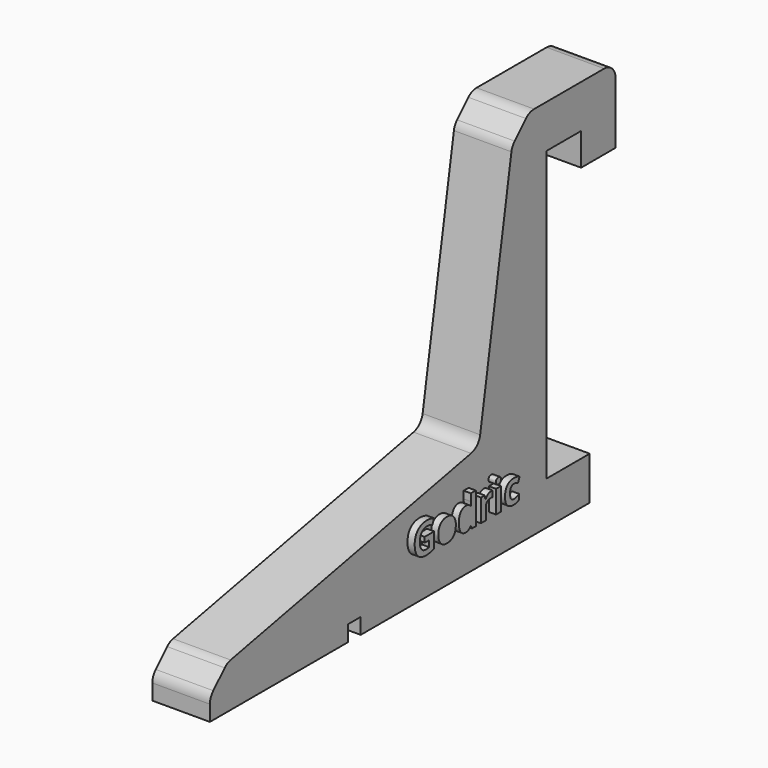
from build123d import *

# Parameters (mm, degrees)
F0_W         = 0.8586518646
F0_H         = 3.1480898372
F1_DEPTH     = 8
F0_TEXT_SIZE = 5.766392375
F2_DEPTH     = 9
F3_R         = 2


# Not quite as in the source:
# - Text() gives the source's letters only with a copy of the font that has no kerning and outlines rounded to 1/6400 em; it was checked with that copy


with BuildPart() as f1:
    # F0 (on Right) → F1 (new body)
    with BuildSketch(Plane.YZ):
        Polygon((0, -40.1), (0, 0), (6, 0), (6, -3.5), (6, -4.5), (7, -4.5), (11, -4.5), (12, -4.5), (12, -3.5), (12, 6), (-3, 6), (-6, 3), (-11.7668367097, -31.4132497789), (-55.5, -40.1), (-58.5, -43.1), (-58.5, -46.1), (-39.6, -46.1), (-37.4, -46.1), (-34.5, -46.1), (-34.5, -43.9), (-32.3, -43.9), (-32.3, -46.1), (7.5, -46.1), (7.5, -40.1), (6, -40.1), align=None)
        with BuildLine():
            Line((-22.4218487444, -38.5151430957), (-22.4218487444, -37.7880370571))
            Line((-22.4218487444, -37.7880370571), (-20.7883379044, -37.7880370571))
            Line((-20.7883379044, -37.7880370571), (-20.7883379044, -39.9225032347))
            add(Edge.make_bspline(
                [(-20.7883379044, -39.9225032347), (-21.185678379, -40.0522470631), (-21.5361669155, -40.104504994)],
                knots=[0, 0, 0, 1, 1, 1], degree=2))
            add(Edge.make_bspline(
                [(-21.5361669155, -40.104504994), (-21.8866554521, -40.1567629249), (-22.2524609684, -40.1567629249)],
                knots=[0, 0, 0, 1, 1, 1], degree=2))
            add(Edge.make_bspline(
                [(-22.2524609684, -40.1567629249), (-23.1840937364, -40.1567629249), (-23.6755885865, -39.6089556493)],
                knots=[0, 0, 0, 1, 1, 1], degree=2))
            add(Edge.make_bspline(
                [(-23.6755885865, -39.6089556493), (-24.1670834366, -39.0611483737), (-24.1670834366, -38.0358117295)],
                knots=[0, 0, 0, 1, 1, 1], degree=2))
            add(Edge.make_bspline(
                [(-24.1670834366, -38.0358117295), (-24.1670834366, -37.0393070472), (-23.5967511908, -36.4820392841)],
                knots=[0, 0, 0, 1, 1, 1], degree=2))
            add(Edge.make_bspline(
                [(-23.5967511908, -36.4820392841), (-23.0264189449, -35.924771521), (-22.0163992805, -35.924771521)],
                knots=[0, 0, 0, 1, 1, 1], degree=2))
            add(Edge.make_bspline(
                [(-22.0163992805, -35.924771521), (-21.3820961192, -35.924771521), (-20.7937438972, -36.1779521862)],
                knots=[0, 0, 0, 1, 1, 1], degree=2))
            Line((-20.7937438972, -36.1779521862), (-21.0838655136, -36.8762262628))
            add(Edge.make_bspline(
                [(-21.0838655136, -36.8762262628), (-21.5343649179, -36.6509765607), (-22.0218052733, -36.6509765607)],
                knots=[0, 0, 0, 1, 1, 1], degree=2))
            add(Edge.make_bspline(
                [(-22.0218052733, -36.6509765607), (-22.5876325251, -36.6509765607), (-22.9282100748, -37.0311980579)],
                knots=[0, 0, 0, 1, 1, 1], degree=2))
            add(Edge.make_bspline(
                [(-22.9282100748, -37.0311980579), (-23.2687876245, -37.4114195551), (-23.2687876245, -38.0529307069)],
                knots=[0, 0, 0, 1, 1, 1], degree=2))
            add(Edge.make_bspline(
                [(-23.2687876245, -38.0529307069), (-23.2687876245, -38.7232738205), (-22.9944334872, -39.0764653534)],
                knots=[0, 0, 0, 1, 1, 1], degree=2))
            add(Edge.make_bspline(
                [(-22.9944334872, -39.0764653534), (-22.72007935, -39.4296568864), (-22.1965990422, -39.4296568864)],
                knots=[0, 0, 0, 1, 1, 1], degree=2))
            add(Edge.make_bspline(
                [(-22.1965990422, -39.4296568864), (-21.9226954044, -39.4296568864), (-21.6415837761, -39.3737949603)],
                knots=[0, 0, 0, 1, 1, 1], degree=2))
            Line((-21.6415837761, -39.3737949603), (-21.6415837761, -38.5151430957))
            Line((-21.6415837761, -38.5151430957), (-22.4218487444, -38.5151430957))
        make_face(mode=Mode.SUBTRACT)
        with BuildLine():
            add(Edge.make_bspline(
                [(-17.2014616473, -37.6560407317), (-17.0158558928, -38.0249997438), (-17.0158558928, -38.5205490885)],
                knots=[0, 0, 0, 1, 1, 1], degree=2))
            add(Edge.make_bspline(
                [(-17.0158558928, -38.5205490885), (-17.0158558928, -39.2891010723), (-17.4213053566, -39.7229319986)],
                knots=[0, 0, 0, 1, 1, 1], degree=2))
            add(Edge.make_bspline(
                [(-17.4213053566, -39.7229319986), (-17.8267548205, -40.1567629249), (-18.5502568638, -40.1567629249)],
                knots=[0, 0, 0, 1, 1, 1], degree=2))
            add(Edge.make_bspline(
                [(-18.5502568638, -40.1567629249), (-19.0034592645, -40.1567629249), (-19.3498933064, -39.9580926876)],
                knots=[0, 0, 0, 1, 1, 1], degree=2))
            add(Edge.make_bspline(
                [(-19.3498933064, -39.9580926876), (-19.6963273484, -39.7594224503), (-19.8819331029, -39.3877604418)],
                knots=[0, 0, 0, 1, 1, 1], degree=2))
            add(Edge.make_bspline(
                [(-19.8819331029, -39.3877604418), (-20.0675388575, -39.0160984333), (-20.0675388575, -38.5205490885)],
                knots=[0, 0, 0, 1, 1, 1], degree=2))
            add(Edge.make_bspline(
                [(-20.0675388575, -38.5205490885), (-20.0675388575, -37.7492941084), (-19.6652428895, -37.3213196743)],
                knots=[0, 0, 0, 1, 1, 1], degree=2))
            add(Edge.make_bspline(
                [(-19.6652428895, -37.3213196743), (-19.2629469214, -36.8933452402), (-18.5331378865, -36.8933452402)],
                knots=[0, 0, 0, 1, 1, 1], degree=2))
            add(Edge.make_bspline(
                [(-18.5331378865, -36.8933452402), (-18.0799354857, -36.8933452402), (-17.7335014438, -37.0902134799)],
                knots=[0, 0, 0, 1, 1, 1], degree=2))
            add(Edge.make_bspline(
                [(-17.7335014438, -37.0902134799), (-17.3870674019, -37.2870817196), (-17.2014616473, -37.6560407317)],
                knots=[0, 0, 0, 1, 1, 1], degree=2))
        make_face(mode=Mode.SUBTRACT)
        with BuildLine():
            add(Edge.make_bspline(
                [(-14.41647433, -39.6918475397), (-14.7092989428, -40.1567629249), (-15.3093641493, -40.1567629249)],
                knots=[0, 0, 0, 1, 1, 1], degree=2))
            add(Edge.make_bspline(
                [(-15.3093641493, -40.1567629249), (-15.8634784166, -40.1567629249), (-16.1801794978, -39.725634995)],
                knots=[0, 0, 0, 1, 1, 1], degree=2))
            add(Edge.make_bspline(
                [(-16.1801794978, -39.725634995), (-16.496880579, -39.2945070651), (-16.496880579, -38.5313610742)],
                knots=[0, 0, 0, 1, 1, 1], degree=2))
            add(Edge.make_bspline(
                [(-16.496880579, -38.5313610742), (-16.496880579, -37.7574030976), (-16.1747735049, -37.3253741689)],
                knots=[0, 0, 0, 1, 1, 1], degree=2))
            add(Edge.make_bspline(
                [(-16.1747735049, -37.3253741689), (-15.8526664309, -36.8933452402), (-15.2868391791, -36.8933452402)],
                knots=[0, 0, 0, 1, 1, 1], degree=2))
            add(Edge.make_bspline(
                [(-15.2868391791, -36.8933452402), (-14.6921799654, -36.8933452402), (-14.3795333788, -37.3546566302)],
                knots=[0, 0, 0, 1, 1, 1], degree=2))
            Line((-14.3795333788, -37.3546566302), (-14.3516024157, -37.3546566302))
            add(Edge.make_bspline(
                [(-14.3516024157, -37.3546566302), (-14.41647433, -37.002366096), (-14.41647433, -36.7266604606)],
                knots=[0, 0, 0, 1, 1, 1], degree=2))
            Line((-14.41647433, -36.7266604606), (-14.41647433, -35.7184427938))
            Line((-14.41647433, -35.7184427938), (-13.5551194689, -35.7184427938))
            Line((-13.5551194689, -35.7184427938), (-13.5551194689, -40.1))
            Line((-13.5551194689, -40.1), (-14.213749598, -40.1))
            Line((-14.213749598, -40.1), (-14.3795333788, -39.6918475397))
            Line((-14.3795333788, -39.6918475397), (-14.41647433, -39.6918475397))
        make_face(mode=Mode.SUBTRACT)
        with BuildLine():
            add(Edge.make_bspline(
                [(-11.4418267634, -37.0550745263), (-11.1927005928, -36.8933452402), (-10.89987598, -36.8933452402)],
                knots=[0, 0, 0, 1, 1, 1], degree=2))
            add(Edge.make_bspline(
                [(-10.89987598, -36.8933452402), (-10.7250822111, -36.8933452402), (-10.6097543636, -36.9185732068)],
                knots=[0, 0, 0, 1, 1, 1], degree=2))
            Line((-10.6097543636, -36.9185732068), (-10.6746262779, -37.7231651429))
            add(Edge.make_bspline(
                [(-10.6746262779, -37.7231651429), (-10.7791421397, -37.6952341798), (-10.9278069431, -37.6952341798)],
                knots=[0, 0, 0, 1, 1, 1], degree=2))
            add(Edge.make_bspline(
                [(-10.9278069431, -37.6952341798), (-11.3386623998, -37.6952341798), (-11.568417096, -37.9065184005)],
                knots=[0, 0, 0, 1, 1, 1], degree=2))
            add(Edge.make_bspline(
                [(-11.568417096, -37.9065184005), (-11.7981717922, -38.1178026211), (-11.7981717922, -38.4980241183)],
                knots=[0, 0, 0, 1, 1, 1], degree=2))
            Line((-11.7981717922, -38.4980241183), (-11.7981717922, -40.1))
            Line((-11.7981717922, -40.1), (-12.6568236568, -40.1))
            Line((-12.6568236568, -40.1), (-12.6568236568, -36.9519101628))
            Line((-12.6568236568, -36.9519101628), (-12.006302517, -36.9519101628))
            Line((-12.006302517, -36.9519101628), (-11.879261685, -37.4816974622))
            Line((-11.879261685, -37.4816974622), (-11.8378157398, -37.4816974622))
            add(Edge.make_bspline(
                [(-11.8378157398, -37.4816974622), (-11.690952934, -37.2168038125), (-11.4418267634, -37.0550745263)],
                knots=[0, 0, 0, 1, 1, 1], degree=2))
        make_face(mode=Mode.SUBTRACT)
        with Locations((-9.6091951867, -38.5259550814)):
            Rectangle(F0_W, F0_H, mode=Mode.SUBTRACT)
        with BuildLine():
            add(Edge.make_bspline(
                [(-6.4642588453, -40.1058564923), (-6.6768945641, -40.1567629249), (-7.0003531364, -40.1567629249)],
                knots=[0, 0, 0, 1, 1, 1], degree=2))
            add(Edge.make_bspline(
                [(-7.0003531364, -40.1567629249), (-8.4698821932, -40.1567629249), (-8.4698821932, -38.5430740587)],
                knots=[0, 0, 0, 1, 1, 1], degree=2))
            add(Edge.make_bspline(
                [(-8.4698821932, -38.5430740587), (-8.4698821932, -37.7402841203), (-8.0702892216, -37.3168146802)],
                knots=[0, 0, 0, 1, 1, 1], degree=2))
            add(Edge.make_bspline(
                [(-8.0702892216, -37.3168146802), (-7.67069625, -36.8933452402), (-6.9246692365, -36.8933452402)],
                knots=[0, 0, 0, 1, 1, 1], degree=2))
            add(Edge.make_bspline(
                [(-6.9246692365, -36.8933452402), (-6.3786639585, -36.8933452402), (-5.9443825327, -37.1068819578)],
                knots=[0, 0, 0, 1, 1, 1], degree=2))
            Line((-5.9443825327, -37.1068819578), (-6.1984641967, -37.7718190786))
            add(Edge.make_bspline(
                [(-6.1984641967, -37.7718190786), (-6.4011889287, -37.689828187), (-6.5755321981, -37.6375702561)],
                knots=[0, 0, 0, 1, 1, 1], degree=2))
            add(Edge.make_bspline(
                [(-6.5755321981, -37.6375702561), (-6.7498754676, -37.5853123252), (-6.9246692365, -37.5853123252)],
                knots=[0, 0, 0, 1, 1, 1], degree=2))
            add(Edge.make_bspline(
                [(-6.9246692365, -37.5853123252), (-7.5950123501, -37.5853123252), (-7.5950123501, -38.5376680659)],
                knots=[0, 0, 0, 1, 1, 1], degree=2))
            add(Edge.make_bspline(
                [(-7.5950123501, -38.5376680659), (-7.5950123501, -39.4611918447), (-6.9246692365, -39.4611918447)],
                knots=[0, 0, 0, 1, 1, 1], degree=2))
            add(Edge.make_bspline(
                [(-6.9246692365, -39.4611918447), (-6.6768945641, -39.4611918447), (-6.4656103435, -39.3949684323)],
                knots=[0, 0, 0, 1, 1, 1], degree=2))
            add(Edge.make_bspline(
                [(-6.4656103435, -39.3949684323), (-6.2543261229, -39.3287450198), (-6.0434924017, -39.1872882069)],
                knots=[0, 0, 0, 1, 1, 1], degree=2))
            Line((-6.0434924017, -39.1872882069), (-6.0434924017, -39.9225032347))
            add(Edge.make_bspline(
                [(-6.0434924017, -39.9225032347), (-6.2516231264, -40.0549500596), (-6.4642588453, -40.1058564923)],
                knots=[0, 0, 0, 1, 1, 1], degree=2))
        make_face(mode=Mode.SUBTRACT)
        with BuildLine():
            add(Edge.make_bspline(
                [(-9.6078436885, -36.5608766798), (-10.0754620701, -36.5608766798), (-10.0754620701, -36.1383082386)],
                knots=[0, 0, 0, 1, 1, 1], degree=2))
            add(Edge.make_bspline(
                [(-10.0754620701, -36.1383082386), (-10.0754620701, -35.7184427938), (-9.6078436885, -35.7184427938)],
                knots=[0, 0, 0, 1, 1, 1], degree=2))
            add(Edge.make_bspline(
                [(-9.6078436885, -35.7184427938), (-9.1402253068, -35.7184427938), (-9.1402253068, -36.1383082386)],
                knots=[0, 0, 0, 1, 1, 1], degree=2))
            add(Edge.make_bspline(
                [(-9.1402253068, -36.1383082386), (-9.1402253068, -36.3383299741), (-9.2569046525, -36.449603327)],
                knots=[0, 0, 0, 1, 1, 1], degree=2))
            add(Edge.make_bspline(
                [(-9.2569046525, -36.449603327), (-9.3735839982, -36.5608766798), (-9.6078436885, -36.5608766798)],
                knots=[0, 0, 0, 1, 1, 1], degree=2))
        make_face(mode=Mode.SUBTRACT)
    extrude(amount=F1_DEPTH)

    # F0 (on Right) → F2 (join)
    with BuildSketch(Plane.YZ):
        with BuildLine():
            add(Edge.make_bspline(
                [(-19.0404002157, -37.8177700178), (-19.1926690143, -38.0502277104), (-19.1926690143, -38.5205490885)],
                knots=[0, 0, 0, 1, 1, 1], degree=2))
            add(Edge.make_bspline(
                [(-19.1926690143, -38.5205490885), (-19.1926690143, -38.9881674702), (-19.0390487175, -39.2273826539)],
                knots=[0, 0, 0, 1, 1, 1], degree=2))
            add(Edge.make_bspline(
                [(-19.0390487175, -39.2273826539), (-18.8854284206, -39.4665978376), (-18.5394448781, -39.4665978376)],
                knots=[0, 0, 0, 1, 1, 1], degree=2))
            add(Edge.make_bspline(
                [(-18.5394448781, -39.4665978376), (-18.1952633332, -39.4665978376), (-18.0447965322, -39.2287341521)],
                knots=[0, 0, 0, 1, 1, 1], degree=2))
            add(Edge.make_bspline(
                [(-18.0447965322, -39.2287341521), (-17.8943297312, -38.9908704666), (-17.8943297312, -38.5205490885)],
                knots=[0, 0, 0, 1, 1, 1], degree=2))
            add(Edge.make_bspline(
                [(-17.8943297312, -38.5205490885), (-17.8943297312, -38.0529307069), (-18.0461480304, -37.819121516)],
                knots=[0, 0, 0, 1, 1, 1], degree=2))
            add(Edge.make_bspline(
                [(-18.0461480304, -37.819121516), (-18.1979663297, -37.5853123252), (-18.544850871, -37.5853123252)],
                knots=[0, 0, 0, 1, 1, 1], degree=2))
            add(Edge.make_bspline(
                [(-18.544850871, -37.5853123252), (-18.888131417, -37.5853123252), (-19.0404002157, -37.8177700178)],
                knots=[0, 0, 0, 1, 1, 1], degree=2))
        make_face()
        with BuildLine():
            add(Edge.make_bspline(
                [(-15.4670389408, -39.2395461378), (-15.3066611529, -39.4720038304), (-15.0075295484, -39.4720038304)],
                knots=[0, 0, 0, 1, 1, 1], degree=2))
            add(Edge.make_bspline(
                [(-15.0075295484, -39.4720038304), (-14.6786649833, -39.4720038304), (-14.5250446864, -39.2805415836)],
                knots=[0, 0, 0, 1, 1, 1], degree=2))
            add(Edge.make_bspline(
                [(-14.5250446864, -39.2805415836), (-14.3714243895, -39.0890793368), (-14.3570084086, -38.6304709432)],
                knots=[0, 0, 0, 1, 1, 1], degree=2))
            Line((-14.3570084086, -38.6304709432), (-14.3570084086, -38.5376680659))
            add(Edge.make_bspline(
                [(-14.3570084086, -38.5376680659), (-14.3570084086, -38.0304057366), (-14.5133317019, -37.8110125268)],
                knots=[0, 0, 0, 1, 1, 1], degree=2))
            add(Edge.make_bspline(
                [(-14.5133317019, -37.8110125268), (-14.6696549952, -37.5916193169), (-15.0219455293, -37.5916193169)],
                knots=[0, 0, 0, 1, 1, 1], degree=2))
            add(Edge.make_bspline(
                [(-15.0219455293, -37.5916193169), (-15.3093641493, -37.5916193169), (-15.468390439, -37.8348889952)],
                knots=[0, 0, 0, 1, 1, 1], degree=2))
            add(Edge.make_bspline(
                [(-15.468390439, -37.8348889952), (-15.6274167287, -38.0781586735), (-15.6274167287, -38.5430740587)],
                knots=[0, 0, 0, 1, 1, 1], degree=2))
            add(Edge.make_bspline(
                [(-15.6274167287, -38.5430740587), (-15.6274167287, -39.0070884452), (-15.4670389408, -39.2395461378)],
                knots=[0, 0, 0, 1, 1, 1], degree=2))
        make_face()
        with Locations((-24.5022549934, -40.1)):
            Text('Godric', F0_TEXT_SIZE, font='Open Sans', font_style=FontStyle.BOLD, text_align=(TextAlign.LEFT, TextAlign.BOTTOM))
    extrude(amount=F2_DEPTH)

    # F3
    f3_edges = [f1.edges().sort_by_distance(p)[0] for p in [
        (4, -58.5, -43.1),
        (4, -55.5, -40.1),
        (4, -11.766837, -31.41325),
        (4, -6, 3),
        (4, -3, 6),
        (4, 12, 6),
    ]]
    fillet(f3_edges, radius=F3_R)


solid = f1.part
